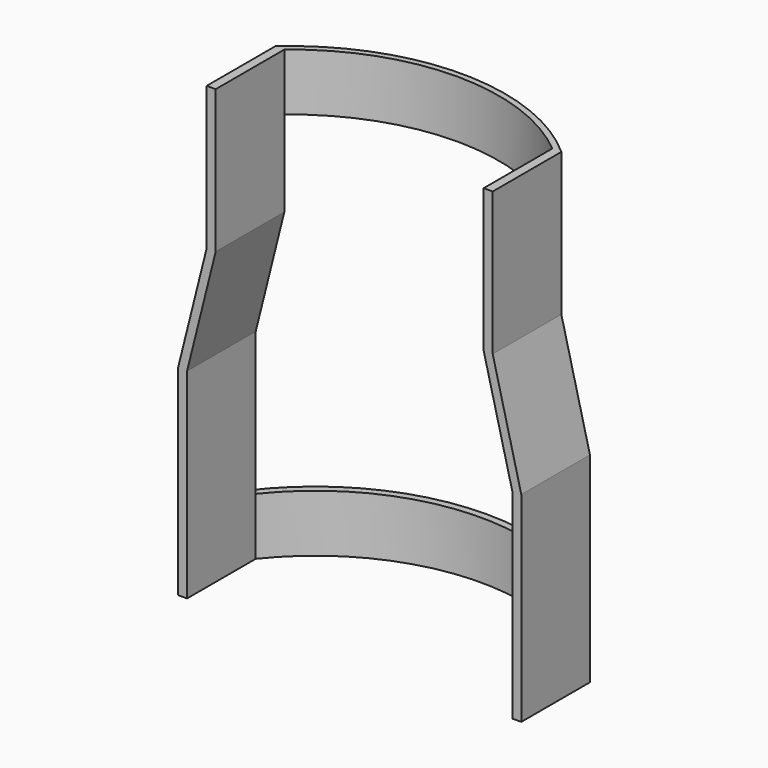
from build123d import *

# Parameters (mm, degrees)
F1_DEPTH = 25.4
F2_DEPTH = 38.1
F4_DEPTH = 38.1
F7_DEPTH = 25.4


# Not quite as in the source:
# - a pattern or mirror of a feature is missing from the dataset's text; its kind, count and spacing are read off the source's solid


with BuildPart() as f1:
    # F0 (on Top) → F1 (new body)
    with BuildSketch(Plane.XY):
        with BuildLine():
            Line((148.3919879557, 0), (152.4, 0))
            ThreePointArc((152.4, 0), (76.2, 38.1), (0, 0))
            Line((0, 0), (4.0080120443, 0))
            ThreePointArc((4.0080120443, 0), (76.2, 34.925), (148.3919879557, 0))
        make_face()
    extrude(amount=F1_DEPTH)

    # F2 (add): faces of the model
    f2_faces = [f1.faces().sort_by_distance(p)[0] for p in [
        (150.3959939779, 0, 12.7),
        (2.0040060221, 0, 12.7),
    ]]
    extrude(f2_faces, amount=F2_DEPTH)

    # F3 (on Front) → F4 (join)
    with BuildSketch(Plane.XZ):
        Polygon((0, 25.4), (4.0080120443, 25.4), (4.0080120443, 88.9), (16.7080120443, 139.7), (16.7080120443, 203.2), (12.7, 203.2), (12.7, 139.7), (0, 88.9), align=None)
    f4 = extrude(amount=F4_DEPTH)

    # F4_copies: F4 across plane
    add(f4.mirror(Plane(origin=(76.2, 0, 0), x_dir=(0, 0, 1), z_dir=(1, 0, 0))))

    # F6 (on face) → F7 (join)
    with BuildSketch(Plane.XY.offset(203.2)):
        with BuildLine():
            ThreePointArc((16.7080120443, 0), (76.2, 21.631021226), (135.6919879557, 0))
            Line((135.6919879557, 0), (139.7, 0))
            ThreePointArc((139.7, 0), (76.2, 24.2548417144), (12.7, 0))
            Line((12.7, 0), (16.7080120443, 0))
        make_face()
    extrude(amount=-F7_DEPTH)


solid = f1.part
